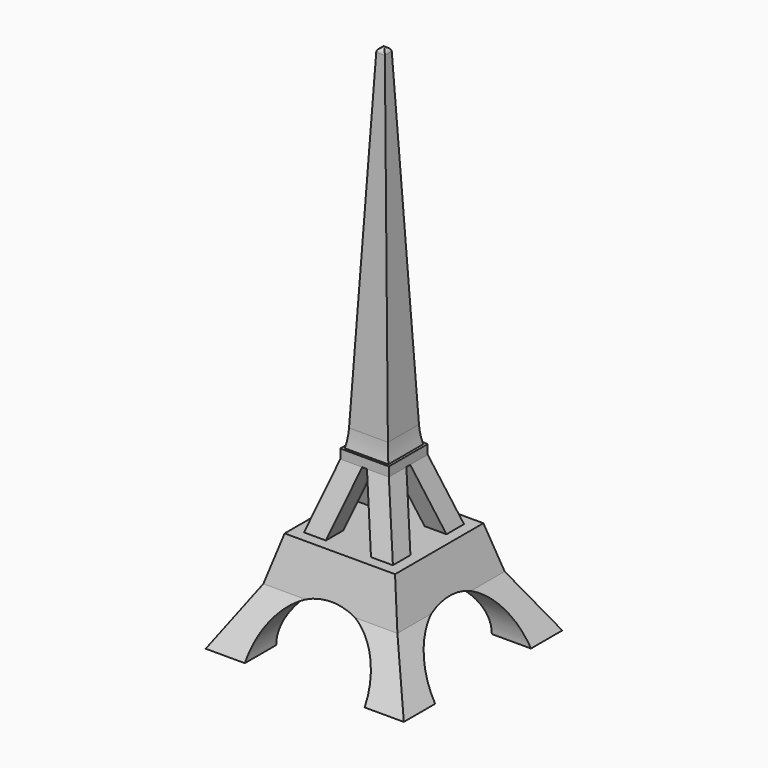
from build123d import *

# Parameters (mm, degrees)
F0_W          = 38
F0_H          = 100
F1_DEPTH      = 38
F3_DEPTH      = 38.001
F4_W          = 59.0429029957
F4_H          = 114.0045975335
F5_DEPTH      = 38.001
F6_T4_DEPTH   = 20.6495370786
F6_T10_DEPTH  = 33.6326816688
F6_T16_DEPTH  = 20.6495370786
F6_S17_R      = 11.4862592402
F6_T18_DEPTH  = 13
F6_T25_DEPTH  = 20.6495370786
F6_T31_DEPTH  = 33.6326816688
F6_T37_DEPTH  = 33.6326816688
F6_T43_DEPTH  = 20.6495370786
F6_T49_DEPTH  = 20.6495370786
F6_S53_R      = 11.4862592402
F6_T54_DEPTH  = 13
F6_T58_DEPTH  = 33.6326816688
F6_T64_DEPTH  = 20.6495370786
F6_T70_DEPTH  = 33.6326816688
F6_T76_DEPTH  = 20.6495370786
F6_T82_DEPTH  = 20.6495370786
F6_S84_R      = 11.4862592402
F6_T85_DEPTH  = 13
F6_T91_DEPTH  = 33.6326816688
F6_T97_DEPTH  = 20.6495370786
F6_T103_DEPTH = 33.6326816688
F6_T109_DEPTH = 20.6495370786
F6_T115_DEPTH = 20.6495370786
F6_S119_R     = 11.4862592402
F6_T120_DEPTH = 13
F6_T124_DEPTH = 33.6326816688
F6_T130_DEPTH = 20.6495370786
F6_T137_DEPTH = 33.6326816688
F6_T143_DEPTH = 33.6326816688
F6_T152_DEPTH = 33.6326816688
F6_T158_DEPTH = 33.6326816688
F6_T167_DEPTH = 33.6326816688
F6_T173_DEPTH = 33.6326816688
F6_T182_DEPTH = 33.6326816688
F6_T188_DEPTH = 33.6326816688


# Not quite as in the source:
# - a fillet or chamfer that OpenCascade refuses, or shapes differently, is made with other operations: its cross-section is extruded or revolved along the edge and cut away or added


with BuildPart() as f1:
    # F0 (on Front) → F1 (new body)
    with BuildSketch(Plane.XZ):
        with Locations((19, 50)):
            Rectangle(F0_W, F0_H)
    extrude(amount=F1_DEPTH)

    # F2 (on face) → F3 (cut, through all)
    with BuildSketch(Plane.XZ.offset(38)):
        with BuildLine():
            ThreePointArc((18.1722940034, 99.2366278339), (18.4188712552, 99.7784903919), (18.9714550646, 100))
            Line((18.9714550646, 100), (0, 100))
            Line((0, 100), (0, 0))
            Line((0, 0), (8.6752314607, 14.7728872032))
            Line((8.6752314607, 14.7728872032), (8.6752314607, 18.7919850665))
            Line((8.6752314607, 18.7919850665), (10.4733575719, 18.7919850665))
            Line((10.4733575719, 18.7919850665), (14.3412563191, 30.8507295043))
            Line((14.3412563191, 30.8507295043), (14.3412563191, 32.6412431896))
            Line((14.3412563191, 32.6412431896), (14.8252512637, 32.6412431896))
            ThreePointArc((14.8252512637, 32.6412431896), (15.1237302322, 34.3327275734), (15.2759763299, 36.0435841545))
            Line((15.2759763299, 36.0435841545), (18.1722940034, 99.2366278339))
        make_face()
        with BuildLine():
            Line((7.5137407598, 0), (30.4862592402, 0))
            ThreePointArc((30.4862592402, 0), (27.1220117992, 8.1220117992), (19, 11.4862592402))
            ThreePointArc((19, 11.4862592402), (10.8779882008, 8.1220117992), (7.5137407598, 0))
        make_face()
        with BuildLine():
            Line((38, 100), (19.0285449354, 100))
            ThreePointArc((19.0285449354, 100), (19.5811287448, 99.7784903919), (19.8277059966, 99.2366278339))
            Line((19.8277059966, 99.2366278339), (22.7240236701, 36.0435841545))
            ThreePointArc((22.7240236701, 36.0435841545), (22.8762697678, 34.3327275734), (23.1747487363, 32.6412431896))
            Line((23.1747487363, 32.6412431896), (23.6587436809, 32.6412431896))
            Line((23.6587436809, 32.6412431896), (23.6587436809, 30.8507295043))
            Line((23.6587436809, 30.8507295043), (27.5266424281, 18.7919850665))
            Line((27.5266424281, 18.7919850665), (29.3247685393, 18.7919850665))
            Line((29.3247685393, 18.7919850665), (29.3247685393, 14.7728872032))
            Line((29.3247685393, 14.7728872032), (38, 0))
            Line((38, 0), (38, 100))
        make_face()
        Polygon((18.5419868585, 30.8507295043), (14.6740881113, 18.7919850665), (23.3259118887, 18.7919850665), (19.4580131415, 30.8507295043), align=None)
    extrude(amount=-F3_DEPTH, mode=Mode.SUBTRACT)

    # F4 (on Right) → F5 (cut, through all)
    with BuildSketch(Plane.YZ):
        with Locations((-17.0494974502, 52.1172431763)):
            Rectangle(F4_W, F4_H)
        with BuildLine():
            Line((-19.0285449354, 100), (-19, 100))
            Line((-19, 100), (-18.9714550646, 100))
            ThreePointArc((-18.9714550646, 100), (-18.4188712552, 99.7784903919), (-18.1722940034, 99.2366278339))
            Line((-18.1722940034, 99.2366278339), (-15.2759763299, 36.0435841545))
            ThreePointArc((-15.2759763299, 36.0435841545), (-15.1237302322, 34.3327275734), (-14.8252512637, 32.6412431896))
            Line((-14.8252512637, 32.6412431896), (-14.3412563191, 32.6412431896))
            Line((-14.3412563191, 32.6412431896), (-14.3412563191, 30.8507295043))
            Line((-14.3412563191, 30.8507295043), (-10.4733575719, 18.7919850665))
            Line((-10.4733575719, 18.7919850665), (-8.6752314607, 18.7919850665))
            Line((-8.6752314607, 18.7919850665), (-8.6752314607, 14.7728872032))
            Line((-8.6752314607, 14.7728872032), (0, 0))
            Line((0, 0), (-7.5137407598, 0))
            ThreePointArc((-7.5137407598, 0), (-10.8779882008, 8.1220117992), (-19, 11.4862592402))
            ThreePointArc((-19, 11.4862592402), (-27.1220117992, 8.1220117992), (-30.4862592402, 0))
            Line((-30.4862592402, 0), (-38, 0))
            Line((-38, 0), (-29.3247685393, 14.7728872032))
            Line((-29.3247685393, 14.7728872032), (-29.3247685393, 18.7919850665))
            Line((-29.3247685393, 18.7919850665), (-27.5266424281, 18.7919850665))
            Line((-27.5266424281, 18.7919850665), (-23.6587436809, 30.8507295043))
            Line((-23.6587436809, 30.8507295043), (-23.6587436809, 32.6412431896))
            Line((-23.6587436809, 32.6412431896), (-23.1747487363, 32.6412431896))
            ThreePointArc((-23.1747487363, 32.6412431896), (-22.8762697678, 34.3327275734), (-22.7240236701, 36.0435841545))
            Line((-22.7240236701, 36.0435841545), (-19.8277059966, 99.2366278339))
            ThreePointArc((-19.8277059966, 99.2366278339), (-19.5811287448, 99.7784903919), (-19.0285449354, 100))
        make_face(mode=Mode.SUBTRACT)
        Polygon((-14.6740881113, 18.7919850665), (-18.5419868585, 30.8507295043), (-19.4580131415, 30.8507295043), (-23.3259118887, 18.7919850665), align=None)
    extrude(amount=F5_DEPTH, mode=Mode.SUBTRACT)

    # F6: chamfer of 5 on 4 edges, made by hand


with BuildPart() as f6_tool2:
    # F6_s3 → F6_t4 (new body)
    with BuildSketch(Plane.XZ.offset(29.3247685393)):
        Polygon((6.1433193707, 10.461342101), (8.6752314607, 19.7728872032), (8.6752314607, 14.7728872032), align=None)
    extrude(amount=-F6_T4_DEPTH)

    split(bisect_by=Plane(origin=(0, -28.2559201757, 16.59300882), x_dir=(1, 0, 0), z_dir=(0, -0.8623090204, 0.506382418)), keep=Keep.TOP)

    split(bisect_by=Plane.XY.offset(18.7919850665), keep=Keep.BOTTOM)


with BuildPart() as f1_1:
    add(f1.part)

    # F6_t1: union F6_tool2
    add(f6_tool2.part)


with BuildPart() as f6_tool8:
    # F6_s9 → F6_t10 (new body)
    with BuildSketch(Plane.XZ.offset(42.3079131295)):
        Polygon((6.1433193707, 10.461342101), (8.6752314607, 19.7728872032), (8.6752314607, 14.7728872032), align=None)
    extrude(amount=-F6_T10_DEPTH)

    split(bisect_by=Plane(origin=(0, -28.2559201757, 16.59300882), x_dir=(1, 0, 0), z_dir=(0, 0.8623090204, -0.506382418)), keep=Keep.TOP)

    split(bisect_by=Plane.XZ.offset(29.3247685393), keep=Keep.TOP)


with BuildPart() as f1_2:
    add(f1_1.part)

    # F6_t7: union F6_tool8
    add(f6_tool8.part)


with BuildPart() as f6_tool14:
    # F6_s15 → F6_t16 (new body)
    with BuildSketch(Plane.XZ.offset(29.3247685393)):
        Polygon((6.1433193707, 10.461342101), (8.6752314607, 19.7728872032), (8.6752314607, 14.7728872032), align=None)
    extrude(amount=-F6_T16_DEPTH)

    # F6_s17 → F6_t18 (cut, symmetric)
    with BuildSketch(Plane.YZ.offset(7.4)):
        with Locations((-19, 0)):
            Circle(F6_S17_R)
    extrude(amount=F6_T18_DEPTH, both=True, mode=Mode.SUBTRACT)

    split(bisect_by=Plane(origin=(0, -28.2559201757, 16.59300882), x_dir=(1, 0, 0), z_dir=(0, 0.8623090204, -0.506382418)), keep=Keep.TOP)

    split(bisect_by=Plane(origin=(0, 0, 0), x_dir=(1, 0, 0), z_dir=(0, -0.8623090204, -0.506382418)), keep=Keep.TOP)

    split(bisect_by=Plane.XY.offset(18.7919850665), keep=Keep.BOTTOM)


with BuildPart() as f1_3:
    add(f1_2.part)

    # F6_t13: union F6_tool14
    add(f6_tool14.part)


with BuildPart() as f6_tool23:
    # F6_s24 → F6_t25 (new body)
    with BuildSketch(Plane.XZ.offset(29.3247685393)):
        Polygon((6.1433193707, 10.461342101), (8.6752314607, 19.7728872032), (8.6752314607, 14.7728872032), align=None)
    extrude(amount=-F6_T25_DEPTH)

    split(bisect_by=Plane(origin=(0, 0, 0), x_dir=(1, 0, 0), z_dir=(0, 0.8623090204, 0.506382418)), keep=Keep.TOP)

    split(bisect_by=Plane.XY.offset(18.7919850665), keep=Keep.BOTTOM)


with BuildPart() as f1_4:
    add(f1_3.part)

    # F6_t22: union F6_tool23
    add(f6_tool23.part)


with BuildPart() as f6_tool29:
    # F6_s30 → F6_t31 (new body)
    with BuildSketch(Plane.XZ.offset(29.3247685393)):
        Polygon((6.1433193707, 10.461342101), (8.6752314607, 19.7728872032), (8.6752314607, 14.7728872032), align=None)
    extrude(amount=-F6_T31_DEPTH)

    split(bisect_by=Plane(origin=(0, 0, 0), x_dir=(1, 0, 0), z_dir=(0, -0.8623090204, -0.506382418)), keep=Keep.TOP)

    split(bisect_by=Plane.XZ.offset(8.6752314607), keep=Keep.BOTTOM)


with BuildPart() as f1_5:
    add(f1_4.part)

    # F6_t28: union F6_tool29
    add(f6_tool29.part)


with BuildPart() as f6_tool35:
    # F6_s36 → F6_t37 (new body)
    with BuildSketch(Plane.YZ.offset(-4.3079131295)):
        Polygon((-29.3247685393, 19.7728872032), (-31.8566806293, 10.461342101), (-29.3247685393, 14.7728872032), align=None)
    extrude(amount=F6_T37_DEPTH)

    split(bisect_by=Plane(origin=(0, 0, 0), x_dir=(0, 1, 0), z_dir=(0.8623090204, 0, -0.506382418)), keep=Keep.TOP)

    split(bisect_by=Plane.YZ.offset(8.6752314607), keep=Keep.BOTTOM)


with BuildPart() as f1_6:
    add(f1_5.part)

    # F6_t34: union F6_tool35
    add(f6_tool35.part)


with BuildPart() as f6_tool41:
    # F6_s42 → F6_t43 (new body)
    with BuildSketch(Plane.YZ.offset(8.6752314607)):
        Polygon((-29.3247685393, 19.7728872032), (-31.8566806293, 10.461342101), (-29.3247685393, 14.7728872032), align=None)
    extrude(amount=F6_T43_DEPTH)

    split(bisect_by=Plane(origin=(0, 0, 0), x_dir=(0, 1, 0), z_dir=(-0.8623090204, 0, 0.506382418)), keep=Keep.TOP)

    split(bisect_by=Plane.XY.offset(18.7919850665), keep=Keep.BOTTOM)


with BuildPart() as f1_7:
    add(f1_6.part)

    # F6_t40: union F6_tool41
    add(f6_tool41.part)


with BuildPart() as f6_tool47:
    # F6_s48 → F6_t49 (new body)
    with BuildSketch(Plane.YZ.offset(8.6752314607)):
        Polygon((-29.3247685393, 19.7728872032), (-31.8566806293, 10.461342101), (-29.3247685393, 14.7728872032), align=None)
    extrude(amount=F6_T49_DEPTH)

    split(bisect_by=Plane(origin=(0, 0, 0), x_dir=(0, 1, 0), z_dir=(0.8623090204, 0, -0.506382418)), keep=Keep.TOP)

    split(bisect_by=Plane.XY.offset(18.7919850665), keep=Keep.BOTTOM)

    split(bisect_by=Plane(origin=(28.2559201757, 0, 16.59300882), x_dir=(0, 1, 0), z_dir=(-0.8623090204, 0, -0.506382418)), keep=Keep.TOP)

    # F6_s53 → F6_t54 (cut, symmetric)
    with BuildSketch(Plane.XZ.offset(30.6)):
        with Locations((19, 0)):
            Circle(F6_S53_R)
    extrude(amount=F6_T54_DEPTH, both=True, mode=Mode.SUBTRACT)


with BuildPart() as f1_8:
    add(f1_7.part)

    # F6_t46: union F6_tool47
    add(f6_tool47.part)


with BuildPart() as f6_tool56:
    # F6_s57 → F6_t58 (new body)
    with BuildSketch(Plane.YZ.offset(8.6752314607)):
        Polygon((-29.3247685393, 19.7728872032), (-31.8566806293, 10.461342101), (-29.3247685393, 14.7728872032), align=None)
    extrude(amount=F6_T58_DEPTH)

    split(bisect_by=Plane.YZ.offset(29.3247685393), keep=Keep.TOP)

    split(bisect_by=Plane(origin=(28.2559201757, 0, 16.59300882), x_dir=(0, 1, 0), z_dir=(-0.8623090204, 0, -0.506382418)), keep=Keep.TOP)


with BuildPart() as f1_9:
    add(f1_8.part)

    # F6_t55: union F6_tool56
    add(f6_tool56.part)


with BuildPart() as f6_tool62:
    # F6_s63 → F6_t64 (new body)
    with BuildSketch(Plane.YZ.offset(8.6752314607)):
        Polygon((-29.3247685393, 19.7728872032), (-31.8566806293, 10.461342101), (-29.3247685393, 14.7728872032), align=None)
    extrude(amount=F6_T64_DEPTH)

    split(bisect_by=Plane.XY.offset(18.7919850665), keep=Keep.BOTTOM)

    split(bisect_by=Plane(origin=(28.2559201757, 0, 16.59300882), x_dir=(0, 1, 0), z_dir=(0.8623090204, 0, 0.506382418)), keep=Keep.TOP)


with BuildPart() as f1_10:
    add(f1_9.part)

    # F6_t61: union F6_tool62
    add(f6_tool62.part)


with BuildPart() as f6_tool68:
    # F6_s69 → F6_t70 (new body)
    with BuildSketch(Plane.XZ.offset(42.3079131295)):
        Polygon((29.3247685393, 19.7728872032), (31.8566806293, 10.461342101), (29.3247685393, 14.7728872032), align=None)
    extrude(amount=-F6_T70_DEPTH)

    split(bisect_by=Plane.XZ.offset(29.3247685393), keep=Keep.TOP)

    split(bisect_by=Plane(origin=(0, -28.2559201757, 16.59300882), x_dir=(1, 0, 0), z_dir=(0, 0.8623090204, -0.506382418)), keep=Keep.TOP)


with BuildPart() as f1_11:
    add(f1_10.part)

    # F6_t67: union F6_tool68
    add(f6_tool68.part)


with BuildPart() as f6_tool74:
    # F6_s75 → F6_t76 (new body)
    with BuildSketch(Plane.XZ.offset(29.3247685393)):
        Polygon((29.3247685393, 19.7728872032), (31.8566806293, 10.461342101), (29.3247685393, 14.7728872032), align=None)
    extrude(amount=-F6_T76_DEPTH)

    split(bisect_by=Plane.XY.offset(18.7919850665), keep=Keep.BOTTOM)

    split(bisect_by=Plane(origin=(0, -28.2559201757, 16.59300882), x_dir=(1, 0, 0), z_dir=(0, -0.8623090204, 0.506382418)), keep=Keep.TOP)


with BuildPart() as f1_12:
    add(f1_11.part)

    # F6_t73: union F6_tool74
    add(f6_tool74.part)


with BuildPart() as f6_tool80:
    # F6_s81 → F6_t82 (new body)
    with BuildSketch(Plane.XZ.offset(29.3247685393)):
        Polygon((29.3247685393, 19.7728872032), (31.8566806293, 10.461342101), (29.3247685393, 14.7728872032), align=None)
    extrude(amount=-F6_T82_DEPTH)

    split(bisect_by=Plane.XY.offset(18.7919850665), keep=Keep.BOTTOM)

    # F6_s84 → F6_t85 (cut, symmetric)
    with BuildSketch(Plane.YZ.offset(30.6)):
        with Locations((-19, 0)):
            Circle(F6_S84_R)
    extrude(amount=F6_T85_DEPTH, both=True, mode=Mode.SUBTRACT)

    split(bisect_by=Plane(origin=(0, 0, 0), x_dir=(1, 0, 0), z_dir=(0, -0.8623090204, -0.506382418)), keep=Keep.TOP)

    split(bisect_by=Plane(origin=(0, -28.2559201757, 16.59300882), x_dir=(1, 0, 0), z_dir=(0, 0.8623090204, -0.506382418)), keep=Keep.TOP)


with BuildPart() as f1_13:
    add(f1_12.part)

    # F6_t79: union F6_tool80
    add(f6_tool80.part)


with BuildPart() as f6_tool89:
    # F6_s90 → F6_t91 (new body)
    with BuildSketch(Plane.XZ.offset(29.3247685393)):
        Polygon((29.3247685393, 19.7728872032), (31.8566806293, 10.461342101), (29.3247685393, 14.7728872032), align=None)
    extrude(amount=-F6_T91_DEPTH)

    split(bisect_by=Plane.XZ.offset(8.6752314607), keep=Keep.BOTTOM)

    split(bisect_by=Plane(origin=(0, 0, 0), x_dir=(1, 0, 0), z_dir=(0, -0.8623090204, -0.506382418)), keep=Keep.TOP)


with BuildPart() as f1_14:
    add(f1_13.part)

    # F6_t88: union F6_tool89
    add(f6_tool89.part)


with BuildPart() as f6_tool95:
    # F6_s96 → F6_t97 (new body)
    with BuildSketch(Plane.XZ.offset(29.3247685393)):
        Polygon((29.3247685393, 19.7728872032), (31.8566806293, 10.461342101), (29.3247685393, 14.7728872032), align=None)
    extrude(amount=-F6_T97_DEPTH)

    split(bisect_by=Plane.XY.offset(18.7919850665), keep=Keep.BOTTOM)

    split(bisect_by=Plane(origin=(0, 0, 0), x_dir=(1, 0, 0), z_dir=(0, 0.8623090204, 0.506382418)), keep=Keep.TOP)


with BuildPart() as f1_15:
    add(f1_14.part)

    # F6_t94: union F6_tool95
    add(f6_tool95.part)


with BuildPart() as f6_tool101:
    # F6_s102 → F6_t103 (new body)
    with BuildSketch(Plane.YZ.offset(-4.3079131295)):
        Polygon((-8.6752314607, 19.7728872032), (-6.1433193707, 10.461342101), (-8.6752314607, 14.7728872032), align=None)
    extrude(amount=F6_T103_DEPTH)

    split(bisect_by=Plane(origin=(0, 0, 0), x_dir=(0, 1, 0), z_dir=(0.8623090204, 0, -0.506382418)), keep=Keep.TOP)

    split(bisect_by=Plane.YZ.offset(8.6752314607), keep=Keep.BOTTOM)


with BuildPart() as f1_16:
    add(f1_15.part)

    # F6_t100: union F6_tool101
    add(f6_tool101.part)


with BuildPart() as f6_tool107:
    # F6_s108 → F6_t109 (new body)
    with BuildSketch(Plane.YZ.offset(8.6752314607)):
        Polygon((-8.6752314607, 19.7728872032), (-6.1433193707, 10.461342101), (-8.6752314607, 14.7728872032), align=None)
    extrude(amount=F6_T109_DEPTH)

    split(bisect_by=Plane(origin=(0, 0, 0), x_dir=(0, 1, 0), z_dir=(-0.8623090204, 0, 0.506382418)), keep=Keep.TOP)

    split(bisect_by=Plane.XY.offset(18.7919850665), keep=Keep.BOTTOM)


with BuildPart() as f1_17:
    add(f1_16.part)

    # F6_t106: union F6_tool107
    add(f6_tool107.part)


with BuildPart() as f6_tool113:
    # F6_s114 → F6_t115 (new body)
    with BuildSketch(Plane.YZ.offset(8.6752314607)):
        Polygon((-8.6752314607, 19.7728872032), (-6.1433193707, 10.461342101), (-8.6752314607, 14.7728872032), align=None)
    extrude(amount=F6_T115_DEPTH)

    split(bisect_by=Plane(origin=(0, 0, 0), x_dir=(0, 1, 0), z_dir=(0.8623090204, 0, -0.506382418)), keep=Keep.TOP)

    split(bisect_by=Plane.XY.offset(18.7919850665), keep=Keep.BOTTOM)

    split(bisect_by=Plane(origin=(28.2559201757, 0, 16.59300882), x_dir=(0, 1, 0), z_dir=(-0.8623090204, 0, -0.506382418)), keep=Keep.TOP)

    # F6_s119 → F6_t120 (cut, symmetric)
    with BuildSketch(Plane.XZ.offset(7.4)):
        with Locations((19, 0)):
            Circle(F6_S119_R)
    extrude(amount=F6_T120_DEPTH, both=True, mode=Mode.SUBTRACT)


with BuildPart() as f1_18:
    add(f1_17.part)

    # F6_t112: union F6_tool113
    add(f6_tool113.part)


with BuildPart() as f6_tool122:
    # F6_s123 → F6_t124 (new body)
    with BuildSketch(Plane.YZ.offset(8.6752314607)):
        Polygon((-8.6752314607, 19.7728872032), (-6.1433193707, 10.461342101), (-8.6752314607, 14.7728872032), align=None)
    extrude(amount=F6_T124_DEPTH)

    split(bisect_by=Plane.YZ.offset(29.3247685393), keep=Keep.TOP)

    split(bisect_by=Plane(origin=(28.2559201757, 0, 16.59300882), x_dir=(0, 1, 0), z_dir=(-0.8623090204, 0, -0.506382418)), keep=Keep.TOP)


with BuildPart() as f1_19:
    add(f1_18.part)

    # F6_t121: union F6_tool122
    add(f6_tool122.part)


with BuildPart() as f6_tool128:
    # F6_s129 → F6_t130 (new body)
    with BuildSketch(Plane.YZ.offset(8.6752314607)):
        Polygon((-8.6752314607, 19.7728872032), (-6.1433193707, 10.461342101), (-8.6752314607, 14.7728872032), align=None)
    extrude(amount=F6_T130_DEPTH)

    split(bisect_by=Plane.XY.offset(18.7919850665), keep=Keep.BOTTOM)

    split(bisect_by=Plane(origin=(28.2559201757, 0, 16.59300882), x_dir=(0, 1, 0), z_dir=(0.8623090204, 0, 0.506382418)), keep=Keep.TOP)


with BuildPart() as f1_20:
    add(f1_19.part)

    # F6_t127: union F6_tool128
    add(f6_tool128.part)


with BuildPart() as f6_tool135:
    # F6_s136 → F6_t137 (new body)
    with BuildSketch(Plane.XZ.offset(42.3079131295)):
        Polygon((6.1433193707, 10.461342101), (8.6752314607, 19.7728872032), (8.6752314607, 14.7728872032), align=None)
    extrude(amount=-F6_T137_DEPTH)

    split(bisect_by=Plane(origin=(0, -28.2559201757, 16.59300882), x_dir=(1, 0, 0), z_dir=(0, -0.8623090204, 0.506382418)), keep=Keep.TOP)

    split(bisect_by=Plane.XZ.offset(29.3247685393), keep=Keep.TOP)

    split(bisect_by=Plane.XY.offset(18.7919850665), keep=Keep.BOTTOM)


with BuildPart() as f6_tool141:
    # F6_s142 → F6_t143 (new body)
    with BuildSketch(Plane.YZ.offset(-4.3079131295)):
        Polygon((-29.3247685393, 19.7728872032), (-31.8566806293, 10.461342101), (-29.3247685393, 14.7728872032), align=None)
    extrude(amount=F6_T143_DEPTH)

    split(bisect_by=Plane(origin=(0, 0, 0), x_dir=(0, 1, 0), z_dir=(-0.8623090204, 0, 0.506382418)), keep=Keep.TOP)

    split(bisect_by=Plane.YZ.offset(8.6752314607), keep=Keep.BOTTOM)

    split(bisect_by=Plane.XY.offset(18.7919850665), keep=Keep.BOTTOM)


with BuildPart() as f6_tool135_1:
    add(f6_tool135.part)

    # F6_t147: intersect F6_tool141
    add(f6_tool141.part, mode=Mode.INTERSECT)


with BuildPart() as f1_21:
    add(f1_20.part)

    # F6_t133: union F6_tool135
    add(f6_tool135_1.part)


with BuildPart() as f6_tool150:
    # F6_s151 → F6_t152 (new body)
    with BuildSketch(Plane.XZ.offset(29.3247685393)):
        Polygon((6.1433193707, 10.461342101), (8.6752314607, 19.7728872032), (8.6752314607, 14.7728872032), align=None)
    extrude(amount=-F6_T152_DEPTH)

    split(bisect_by=Plane(origin=(0, 0, 0), x_dir=(1, 0, 0), z_dir=(0, 0.8623090204, 0.506382418)), keep=Keep.TOP)

    split(bisect_by=Plane.XZ.offset(8.6752314607), keep=Keep.BOTTOM)

    split(bisect_by=Plane.XY.offset(18.7919850665), keep=Keep.BOTTOM)


with BuildPart() as f6_tool156:
    # F6_s157 → F6_t158 (new body)
    with BuildSketch(Plane.YZ.offset(-4.3079131295)):
        Polygon((-8.6752314607, 19.7728872032), (-6.1433193707, 10.461342101), (-8.6752314607, 14.7728872032), align=None)
    extrude(amount=F6_T158_DEPTH)

    split(bisect_by=Plane(origin=(0, 0, 0), x_dir=(0, 1, 0), z_dir=(-0.8623090204, 0, 0.506382418)), keep=Keep.TOP)

    split(bisect_by=Plane.YZ.offset(8.6752314607), keep=Keep.BOTTOM)

    split(bisect_by=Plane.XY.offset(18.7919850665), keep=Keep.BOTTOM)


with BuildPart() as f6_tool150_1:
    add(f6_tool150.part)

    # F6_t162: intersect F6_tool156
    add(f6_tool156.part, mode=Mode.INTERSECT)


with BuildPart() as f1_22:
    add(f1_21.part)

    # F6_t148: union F6_tool150
    add(f6_tool150_1.part)


with BuildPart() as f6_tool165:
    # F6_s166 → F6_t167 (new body)
    with BuildSketch(Plane.XZ.offset(42.3079131295)):
        Polygon((29.3247685393, 19.7728872032), (31.8566806293, 10.461342101), (29.3247685393, 14.7728872032), align=None)
    extrude(amount=-F6_T167_DEPTH)

    split(bisect_by=Plane.XY.offset(18.7919850665), keep=Keep.BOTTOM)

    split(bisect_by=Plane.XZ.offset(29.3247685393), keep=Keep.TOP)

    split(bisect_by=Plane(origin=(0, -28.2559201757, 16.59300882), x_dir=(1, 0, 0), z_dir=(0, -0.8623090204, 0.506382418)), keep=Keep.TOP)


with BuildPart() as f6_tool171:
    # F6_s172 → F6_t173 (new body)
    with BuildSketch(Plane.YZ.offset(8.6752314607)):
        Polygon((-29.3247685393, 19.7728872032), (-31.8566806293, 10.461342101), (-29.3247685393, 14.7728872032), align=None)
    extrude(amount=F6_T173_DEPTH)

    split(bisect_by=Plane.XY.offset(18.7919850665), keep=Keep.BOTTOM)

    split(bisect_by=Plane.YZ.offset(29.3247685393), keep=Keep.TOP)

    split(bisect_by=Plane(origin=(28.2559201757, 0, 16.59300882), x_dir=(0, 1, 0), z_dir=(0.8623090204, 0, 0.506382418)), keep=Keep.TOP)


with BuildPart() as f6_tool165_1:
    add(f6_tool165.part)

    # F6_t177: intersect F6_tool171
    add(f6_tool171.part, mode=Mode.INTERSECT)


with BuildPart() as f1_23:
    add(f1_22.part)

    # F6_t163: union F6_tool165
    add(f6_tool165_1.part)


with BuildPart() as f6_tool180:
    # F6_s181 → F6_t182 (new body)
    with BuildSketch(Plane.XZ.offset(29.3247685393)):
        Polygon((29.3247685393, 19.7728872032), (31.8566806293, 10.461342101), (29.3247685393, 14.7728872032), align=None)
    extrude(amount=-F6_T182_DEPTH)

    split(bisect_by=Plane.XY.offset(18.7919850665), keep=Keep.BOTTOM)

    split(bisect_by=Plane.XZ.offset(8.6752314607), keep=Keep.BOTTOM)

    split(bisect_by=Plane(origin=(0, 0, 0), x_dir=(1, 0, 0), z_dir=(0, 0.8623090204, 0.506382418)), keep=Keep.TOP)


with BuildPart() as f6_tool186:
    # F6_s187 → F6_t188 (new body)
    with BuildSketch(Plane.YZ.offset(8.6752314607)):
        Polygon((-8.6752314607, 19.7728872032), (-6.1433193707, 10.461342101), (-8.6752314607, 14.7728872032), align=None)
    extrude(amount=F6_T188_DEPTH)

    split(bisect_by=Plane.XY.offset(18.7919850665), keep=Keep.BOTTOM)

    split(bisect_by=Plane.YZ.offset(29.3247685393), keep=Keep.TOP)

    split(bisect_by=Plane(origin=(28.2559201757, 0, 16.59300882), x_dir=(0, 1, 0), z_dir=(0.8623090204, 0, 0.506382418)), keep=Keep.TOP)


with BuildPart() as f6_tool180_1:
    add(f6_tool180.part)

    # F6_t192: intersect F6_tool186
    add(f6_tool186.part, mode=Mode.INTERSECT)


with BuildPart() as f1_24:
    add(f1_23.part)

    # F6_t178: union F6_tool180
    add(f6_tool180_1.part)


solid = f1_24.part
